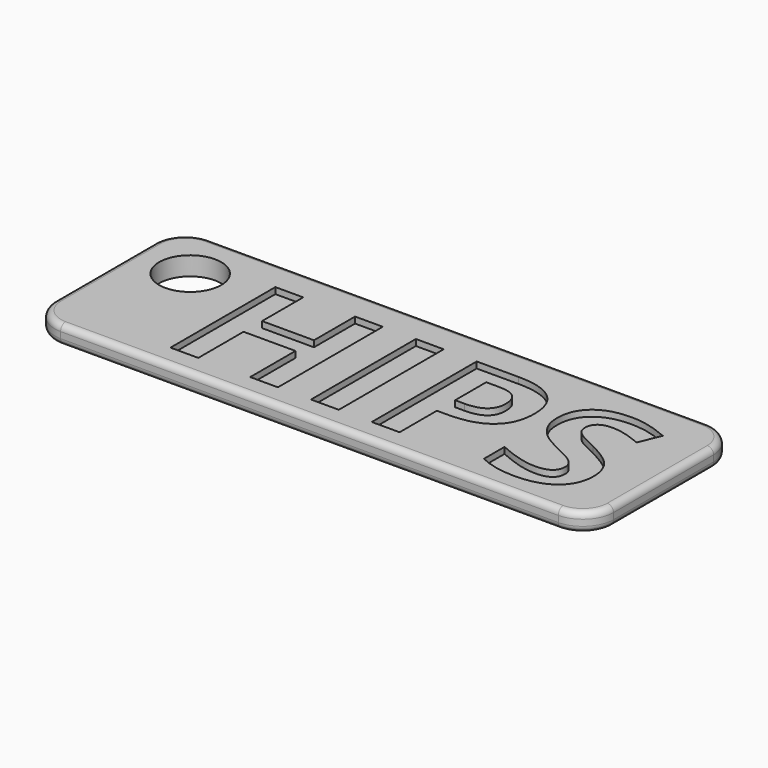
from build123d import *

# Parameters (mm, degrees)
F0_W         = 90
F0_H         = 30
F1_DEPTH     = 3
F2_R         = 1
F3_T1_DEPTH  = 3
F3_T4_ANGLE  = 90
F3_T6_ANGLE  = 90
F3_T8_ANGLE  = 90
F3_T10_ANGLE = 90
F3_T12_ANGLE = 90
F3_T14_ANGLE = 90
F3_T16_ANGLE = 90
F3_T18_ANGLE = 90
F4_R         = 5
F5_DEPTH     = 3
F6_TEXT_SIZE = 29.5612009238
F7_DEPTH     = 1


# Not quite as in the source:
# - a fillet or chamfer that OpenCascade refuses, or shapes differently, is made with other operations: its cross-section is extruded or revolved along the edge and cut away or added
# - Text() gives the source's letters only with a copy of the font that has no kerning and outlines rounded to 1/6400 em; it was checked with that copy


with BuildPart() as f1:
    # F0 (on Top) → F1 (new body)
    with BuildSketch(Plane.XY):
        Rectangle(F0_W, F0_H)
    extrude(amount=F1_DEPTH)

    # F2
    f2_edges = [f1.edges().sort_by_distance(p)[0] for p in [
        (0, 15, 3),
        (-45, 0, 3),
        (0, -15, 3),
        (45, 0, 3),
        (0, 15, 0),
        (-45, 0, 0),
        (0, -15, 0),
        (45, 0, 0),
    ]]
    fillet(f2_edges, radius=F2_R)

    # F3: fillet of radius 5 on 4 edges, made by hand

    # F3_s2 → F3_t1 (cut)
    with BuildSketch(Plane.XY):
        with BuildLine():
            ThreePointArc((45.0004, -9.9990343146), (43.5355339059, -13.5355339059), (39.9990343146, -15.0004))
            Line((39.9990343146, -15.0004), (39.9990343146, -15.5005365685))
            ThreePointArc((39.9990343146, -15.5005365685), (42.4995171573, -15.5001365685), (45, -15.5001365685))
            Line((45, -15.5001365685), (45.5001365685, -15))
            ThreePointArc((45.5001365685, -15), (45.5001365685, -12.4995171573), (45.5005365685, -9.9990343146))
            Line((45.5005365685, -9.9990343146), (45.0004, -9.9990343146))
        make_face()
        with BuildLine():
            ThreePointArc((39.9990343146, 15.0004), (43.5355339059, 13.5355339059), (45.0004, 9.9990343146))
            Line((45.0004, 9.9990343146), (45.5005365685, 9.9990343146))
            ThreePointArc((45.5005365685, 9.9990343146), (45.5001365685, 12.4995171573), (45.5001365685, 15))
            Line((45.5001365685, 15), (45, 15.5001365685))
            ThreePointArc((45, 15.5001365685), (42.4995171573, 15.5001365685), (39.9990343146, 15.5005365685))
            Line((39.9990343146, 15.5005365685), (39.9990343146, 15.0004))
        make_face()
        with BuildLine():
            ThreePointArc((-39.9990343146, 15.0004), (-43.5355339059, 13.5355339059), (-45.0004, 9.9990343146))
            Line((-45.0004, 9.9990343146), (-45.5005365685, 9.9990343146))
            ThreePointArc((-45.5005365685, 9.9990343146), (-45.5001365685, 12.4995171573), (-45.5001365685, 15))
            Line((-45.5001365685, 15), (-45, 15.5001365685))
            ThreePointArc((-45, 15.5001365685), (-42.4995171573, 15.5001365685), (-39.9990343146, 15.5005365685))
            Line((-39.9990343146, 15.5005365685), (-39.9990343146, 15.0004))
        make_face()
        with BuildLine():
            ThreePointArc((-45.0004, -9.9990343146), (-43.5355339059, -13.5355339059), (-39.9990343146, -15.0004))
            Line((-39.9990343146, -15.0004), (-39.9990343146, -15.5005365685))
            ThreePointArc((-39.9990343146, -15.5005365685), (-42.4995171573, -15.5001365685), (-45, -15.5001365685))
            Line((-45, -15.5001365685), (-45.5001365685, -15))
            ThreePointArc((-45.5001365685, -15), (-45.5001365685, -12.4995171573), (-45.5005365685, -9.9990343146))
            Line((-45.5005365685, -9.9990343146), (-45.0004, -9.9990343146))
        make_face()
    extrude(amount=F3_T1_DEPTH, mode=Mode.SUBTRACT)

    # F3_s3 → F3_t4 (revolve, cut)
    with BuildSketch(Plane.YZ.offset(-39.9990343146)):
        with BuildLine():
            ThreePointArc((-14.0004, 0), (-14.7075067812, 0.2928932188), (-15.0004, 1))
            Line((-15.0004, 1), (-15.0004, 0))
            Line((-15.0004, 0), (-14.0004, 0))
        make_face()
    revolve(axis=Axis((-39.9990343146, -9.9990343146, 0), (0, 0, -1)), revolution_arc=F3_T4_ANGLE, mode=Mode.SUBTRACT)

    # F3_s5 → F3_t6 (revolve, cut)
    with BuildSketch(Plane.XZ.offset(9.9990343146)):
        with BuildLine():
            ThreePointArc((-44.0004, 3), (-44.7075067812, 2.7071067812), (-45.0004, 2))
            Line((-45.0004, 2), (-45.0004, 3))
            Line((-45.0004, 3), (-44.0004, 3))
        make_face()
    revolve(axis=Axis((-39.9990343146, -9.9990343146, 3), (0, 0, 1)), revolution_arc=F3_T6_ANGLE, mode=Mode.SUBTRACT)

    # F3_s7 → F3_t8 (revolve, cut)
    with BuildSketch(Plane.XZ.offset(-9.9990343146)):
        with BuildLine():
            ThreePointArc((-44.0004, 0), (-44.7075067812, 0.2928932188), (-45.0004, 1))
            Line((-45.0004, 1), (-45.0004, 0))
            Line((-45.0004, 0), (-44.0004, 0))
        make_face()
    revolve(axis=Axis((-39.9990343146, 9.9990343146, 0), (0, 0, -1)), revolution_arc=F3_T8_ANGLE, mode=Mode.SUBTRACT)

    # F3_s9 → F3_t10 (revolve, cut)
    with BuildSketch(Plane.YZ.offset(-39.9990343146)):
        with BuildLine():
            ThreePointArc((14.0004, 3), (14.7075067812, 2.7071067812), (15.0004, 2))
            Line((15.0004, 2), (15.0004, 3))
            Line((15.0004, 3), (14.0004, 3))
        make_face()
    revolve(axis=Axis((-39.9990343146, 9.9990343146, 3), (0, 0, 1)), revolution_arc=F3_T10_ANGLE, mode=Mode.SUBTRACT)

    # F3_s11 → F3_t12 (revolve, cut)
    with BuildSketch(Plane.YZ.offset(39.9990343146)):
        with BuildLine():
            ThreePointArc((14.0004, 0), (14.7075067812, 0.2928932188), (15.0004, 1))
            Line((15.0004, 1), (15.0004, 0))
            Line((15.0004, 0), (14.0004, 0))
        make_face()
    revolve(axis=Axis((39.9990343146, 9.9990343146, 0), (0, 0, -1)), revolution_arc=F3_T12_ANGLE, mode=Mode.SUBTRACT)

    # F3_s13 → F3_t14 (revolve, cut)
    with BuildSketch(Plane.XZ.offset(-9.9990343146)):
        with BuildLine():
            ThreePointArc((44.0004, 3), (44.7075067812, 2.7071067812), (45.0004, 2))
            Line((45.0004, 2), (45.0004, 3))
            Line((45.0004, 3), (44.0004, 3))
        make_face()
    revolve(axis=Axis((39.9990343146, 9.9990343146, 3), (0, 0, 1)), revolution_arc=F3_T14_ANGLE, mode=Mode.SUBTRACT)

    # F3_s15 → F3_t16 (revolve, cut)
    with BuildSketch(Plane.XZ.offset(9.9990343146)):
        with BuildLine():
            ThreePointArc((44.0004, 0), (44.7075067812, 0.2928932188), (45.0004, 1))
            Line((45.0004, 1), (45.0004, 0))
            Line((45.0004, 0), (44.0004, 0))
        make_face()
    revolve(axis=Axis((39.9990343146, -9.9990343146, 0), (0, 0, -1)), revolution_arc=F3_T16_ANGLE, mode=Mode.SUBTRACT)

    # F3_s17 → F3_t18 (revolve, cut)
    with BuildSketch(Plane.YZ.offset(39.9990343146)):
        with BuildLine():
            ThreePointArc((-14.0004, 3), (-14.7075067812, 2.7071067812), (-15.0004, 2))
            Line((-15.0004, 2), (-15.0004, 3))
            Line((-15.0004, 3), (-14.0004, 3))
        make_face()
    revolve(axis=Axis((39.9990343146, -9.9990343146, 3), (0, 0, 1)), revolution_arc=F3_T18_ANGLE, mode=Mode.SUBTRACT)

    # F4 (on face) → F5 (cut)
    with BuildSketch(Plane.XY.offset(3)):
        with Locations((-36, 6)):
            Circle(F4_R)
    extrude(amount=-F5_DEPTH, mode=Mode.SUBTRACT)

    # F6 (on face) → F7 (cut)
    with BuildSketch(Plane.XY.offset(3)):
        with Locations((-28, -11.2840646651)):
            Text('HIPS', F6_TEXT_SIZE, font='Open Sans', font_style=FontStyle.BOLD, text_align=(TextAlign.LEFT, TextAlign.BOTTOM))
    extrude(amount=-F7_DEPTH, mode=Mode.SUBTRACT)


solid = f1.part
